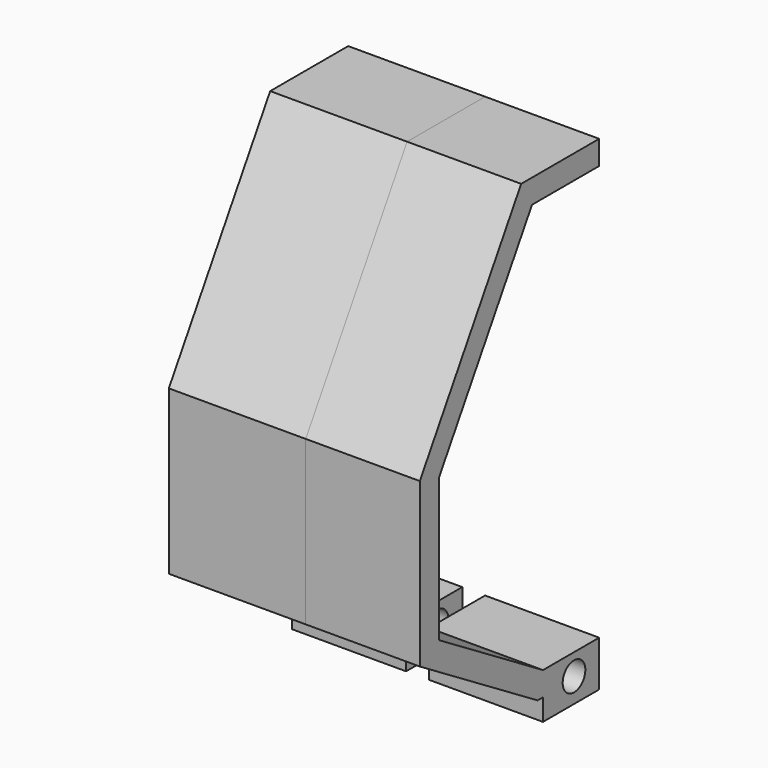
from build123d import *

# Parameters (mm, degrees)
F1_DEPTH = 25.4
F2_DEPTH = 10.16
F3_R     = 3.1528992533
F4_DEPTH = 25.4
F5_DEPTH = 30.48
F6_DEPTH = 5.08
F7_DEPTH = 5.08


with BuildPart() as f1:
    # F0 (on Right) → F1 (new body)
    with BuildSketch(Plane.YZ):
        Polygon((0, 53.3697988007), (0, 58.7037988007), (-21.7103212485, 58.7037988007), (-49.9131307006, 11.9127783076), (-49.9131307006, -24.4350843132), (-44.5791307006, -21.4384287332), (-44.5791307006, 10.4295662253), (-18.6973443152, 53.3697988007), align=None)
        Polygon((-44.5791307006, -21.4384287332), (-49.9131307006, -24.4350843132), (-17.1343572438, -44.4003343582), (0, -44.4003343582), (0, -39.0663343582), (-15.6377889345, -39.0663343582), align=None)
    extrude(amount=F1_DEPTH)

    # F2 (add): a face of the model
    f2_faces = [f1.faces().sort_by_distance(p)[0] for p in [
        (12.7, -7.8188944672, -39.0663343582),
    ]]
    extrude(f2_faces, amount=-F2_DEPTH)

    # F3 (on face) → F4 (cut)
    with BuildSketch(Plane(origin=(0, 0, 0), x_dir=(0, -1, 0), z_dir=(-1, 0, 0))):
        with Locations((7.0027378388, -43.8043549657)):
            Circle(F3_R)
    extrude(amount=-F4_DEPTH, mode=Mode.SUBTRACT)


with BuildPart() as f5:
    # F5 (new): a face of the model
    f5_faces = [f1.part.faces().sort_by_distance(p)[0] for p in [
        (0, -32.6566725698, 32.5135338393),
    ]]
    extrude(f5_faces, amount=F5_DEPTH)

    # F3 (on face) → F6 (cut)
    with BuildSketch(Plane(origin=(0, 0, 0), x_dir=(0, -1, 0), z_dir=(-1, 0, 0))):
        Polygon((0, 53.3697988007), (18.6973443152, 53.3697988007), (44.5791307006, 10.4295662253), (44.5791307006, -21.4384287332), (15.6377889345, -39.0663343582), (0, -39.0663343582), (0, -49.2263343582), (15.6377889345, -49.2263343582), (15.6377889345, -44.4003343582), (17.1343572438, -44.4003343582), (49.9131307006, -24.4350843132), (49.9131307006, 11.9127783076), (21.7103212485, 58.7037988007), (0, 58.7037988007), align=None)
        with Locations((7.0027378388, -43.8043549657)):
            Circle(F3_R, mode=Mode.SUBTRACT)
    extrude(amount=F6_DEPTH, mode=Mode.SUBTRACT)

    # F0 (on Right) → F7 (join)
    with BuildSketch(Plane.YZ):
        Polygon((0, 53.3697988007), (0, 58.7037988007), (-21.7103212485, 58.7037988007), (-49.9131307006, 11.9127783076), (-49.9131307006, -24.4350843132), (-44.5791307006, -21.4384287332), (-44.5791307006, 10.4295662253), (-18.6973443152, 53.3697988007), align=None)
    extrude(amount=-F7_DEPTH)


solid = Compound([f1.part, f5.part])
